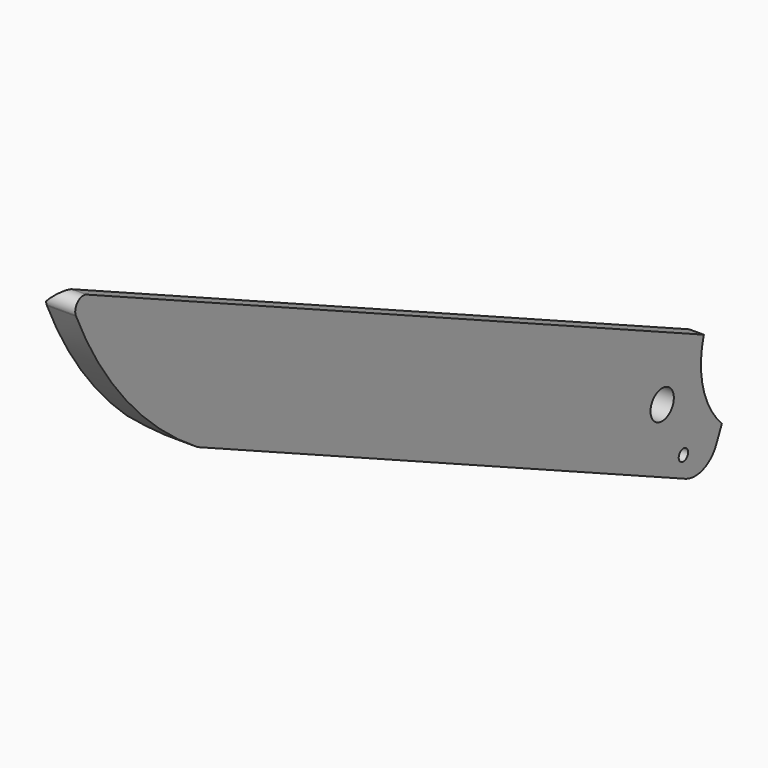
from build123d import *

# Parameters (mm, degrees)
F0_R        = 1
F0_R_2      = 2.5
F1_DEPTH    = 5
F2_T1_DEPTH = 140.5508565822
F2_T3_DEPTH = 158.1494237613


# Not quite as in the source:
# - a fillet or chamfer that OpenCascade refuses, or shapes differently, is made with other operations: its cross-section is extruded or revolved along the edge and cut away or added


with BuildPart() as f1:
    # F0 (on Right) → F1 (new body)
    with BuildSketch(Plane.YZ):
        with BuildLine():
            Line((-238.351838073, 51.1362271676), (-133.7205907933, 3.81650843))
            ThreePointArc((-133.7205907933, 3.81650843), (-129.8957188572, 3.6939702207), (-127.1044783752, 6.3119155052))
            Line((-127.1044783752, 6.3119155052), (-125.8958157643, 8.9844562534))
            ThreePointArc((-125.8958157643, 8.9844562534), (-129.9178817918, 15.9435567205), (-129.7697865993, 23.9799839275))
            Line((-129.7697865993, 23.9799839275), (-224.5101433949, 66.8265250251))
            Line((-224.5101433949, 66.8265250251), (-262.1519725075, 83.8501275596))
            ThreePointArc((-262.1519725075, 83.8501275596), (-264.0478442183, 83.5411975558), (-264.4983908426, 81.6739067294))
            ThreePointArc((-264.4983908426, 81.6739067294), (-264.4532671282, 81.571051598), (-264.4079761186, 81.4682700232))
            ThreePointArc((-264.4079761186, 81.4682700232), (-253.6243159552, 64.3742338109), (-238.351838073, 51.1362271676))
        make_face()
        with Locations((-134.1624917959, 7.5852589493)):
            Circle(F0_R, mode=Mode.SUBTRACT)
        with Locations((-138.7114049438, 17.0487332662)):
            Circle(F0_R_2, mode=Mode.SUBTRACT)
        with BuildLine():
            ThreePointArc((-264.4983908426, 81.6739067294), (-264.4565130864, 81.5696244091), (-264.4079761186, 81.4682700232))
            ThreePointArc((-264.4079761186, 81.4682700232), (-264.4532671282, 81.571051598), (-264.4983908426, 81.6739067294))
        make_face()
    extrude(amount=-F1_DEPTH)

    # F2: chamfer of 2.5 on 2 edges, made by hand

    # F2_s2 → F2_t1 (cut)
    with BuildSketch(Plane(origin=(0, -234.652694271, 106.1222128437), x_dir=(1, 0, 0), z_dir=(0, 0.9111519493, -0.4120705343))):
        Polygon((-2.5, 51.6248961977), (-5, 49.1248961977), (-5, 51.6248961977), align=None)
    extrude(amount=F2_T1_DEPTH, mode=Mode.SUBTRACT)

    # F2_s4 → F2_t3 (cut)
    with BuildSketch(Plane(origin=(0, -110.8801138075, 50.1457827883), x_dir=(1, 0, 0), z_dir=(0, -0.9111519493, 0.4120705343))):
        Polygon((-2.5, -31.6248961977), (-5, -34.1248961977), (-5, -31.6248961977), align=None)
    extrude(amount=F2_T3_DEPTH, mode=Mode.SUBTRACT)


solid = f1.part
